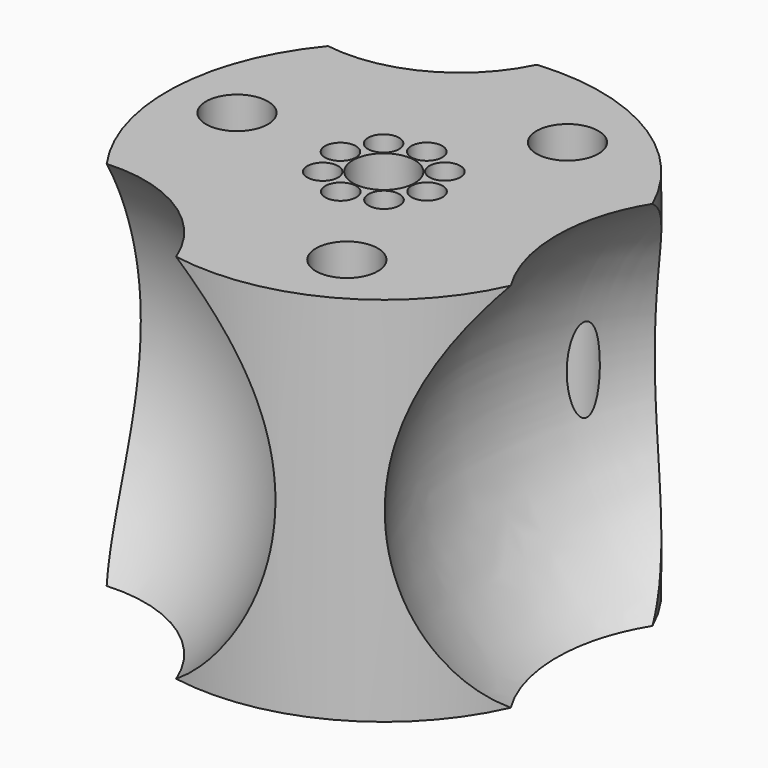
from build123d import *

# Parameters (mm, degrees)
F0_R          = 44.45
F0_R_2        = 16.51
F1_DEPTH      = 38.1
F1_DEPTH_BACK = 38.1
F8_R          = 3.175
F8_R_2        = 1.9685
F9_DEPTH      = 48.26
F10_R         = 6.35
F11_DEPTH     = 7.62
F12_R         = 3.429
F13_DEPTH     = 68.58
F14_R         = 6.35
F15_DEPTH     = 76.2


# Not quite as in the source:
# - a feature names something its author has since deleted; it is built from what else it names


with BuildPart() as f1:
    # F0 (on Top) → F1 (new body, two sides)
    with BuildSketch(Plane.XY) as f1_sk:
        with Locations((-96.7949852347, 47.625)):
            Circle(F0_R)
        with Locations((-96.7949852347, 47.625)):
            Circle(F0_R_2, mode=Mode.SUBTRACT)
        with Locations((-96.7949852347, 47.625)):
            Circle(F0_R_2)
        with BuildLine():
            ThreePointArc((-88.1051627648, 52.1100670498), (-87.4115771175, 50.37826953), (-87.0594782396, 48.5462733292))
            ThreePointArc((-87.0594782396, 48.5462733292), (-85.6757800173, 47.965243489), (-85.103715896, 46.5778145407))
            ThreePointArc((-85.103715896, 46.5778145407), (-85.8323827306, 45.0488259953), (-87.478931514, 44.6517889292))
            ThreePointArc((-87.478931514, 44.6517889292), (-88.2130581693, 42.9367840447), (-89.2595036018, 41.3923956038))
            ThreePointArc((-89.2595036018, 41.3923956038), (-88.839336444, 40.7569162622), (-88.6919210429, 40.0094919292))
            ThreePointArc((-88.6919210429, 40.0094919292), (-90.1000831422, 38.1224270954), (-92.309918185, 38.9351775301))
            ThreePointArc((-92.309918185, 38.9351775301), (-94.0417157047, 38.2415918827), (-95.8737119056, 37.8894930048))
            ThreePointArc((-95.8737119056, 37.8894930048), (-98.0529677671, 35.9450498204), (-99.7681963056, 38.3089462792))
            ThreePointArc((-99.7681963056, 38.3089462792), (-101.48320119, 39.0430729345), (-103.0275896309, 40.089518367))
            ThreePointArc((-103.0275896309, 40.089518367), (-105.9434851899, 40.2555560033), (-105.4848077047, 43.1399329502))
            ThreePointArc((-105.4848077047, 43.1399329502), (-106.178393352, 44.87173047), (-106.5304922299, 46.7037266708))
            ThreePointArc((-106.5304922299, 46.7037266708), (-108.4749354144, 48.8829825323), (-106.1110389555, 50.5982110708))
            ThreePointArc((-106.1110389555, 50.5982110708), (-105.3769123002, 52.3132159553), (-104.3304668677, 53.8576043962))
            ThreePointArc((-104.3304668677, 53.8576043962), (-104.1644292314, 56.7734999551), (-101.2800522845, 56.3148224699))
            ThreePointArc((-101.2800522845, 56.3148224699), (-99.5482547647, 57.0084081173), (-97.7162585639, 57.3605069952))
            ThreePointArc((-97.7162585639, 57.3605069952), (-95.7414309138, 59.3162590358), (-93.7792997754, 57.3477693387))
            ThreePointArc((-93.7792997754, 57.3477693387), (-93.7899471678, 57.1433056087), (-93.8217741639, 56.9410537208))
            ThreePointArc((-93.8217741639, 56.9410537208), (-92.1067692795, 56.2069270655), (-90.5623808386, 55.160481633))
            ThreePointArc((-90.5623808386, 55.160481633), (-88.4202847093, 55.5757742752), (-87.210977164, 53.7595641919))
            ThreePointArc((-87.210977164, 53.7595641919), (-87.4489020941, 52.8214265806), (-88.1051627648, 52.1100670498))
        make_face(mode=Mode.SUBTRACT)
        with BuildLine():
            ThreePointArc((-87.478931514, 44.6517889292), (-89.0293967369, 46.7886116136), (-87.0594782396, 48.5462733292))
            ThreePointArc((-87.0594782396, 48.5462733292), (-87.4115771175, 50.37826953), (-88.1051627648, 52.1100670498))
            ThreePointArc((-88.1051627648, 52.1100670498), (-90.7124690483, 52.524684387), (-90.5623808386, 55.160481633))
            ThreePointArc((-90.5623808386, 55.160481633), (-92.1067692795, 56.2069270655), (-93.8217741639, 56.9410537208))
            ThreePointArc((-93.8217741639, 56.9410537208), (-95.9585968484, 55.3905884978), (-97.7162585639, 57.3605069952))
            ThreePointArc((-97.7162585639, 57.3605069952), (-99.5482547647, 57.0084081173), (-101.2800522845, 56.3148224699))
            ThreePointArc((-101.2800522845, 56.3148224699), (-101.0424845928, 55.8008459714), (-100.9610494266, 55.2405080708))
            ThreePointArc((-100.9610494266, 55.2405080708), (-102.1821250936, 53.4194234719), (-104.3304668677, 53.8576043962))
            ThreePointArc((-104.3304668677, 53.8576043962), (-105.3769123002, 52.3132159553), (-106.1110389555, 50.5982110708))
            ThreePointArc((-106.1110389555, 50.5982110708), (-104.988766028, 49.9120186247), (-104.5492545734, 48.6721854593))
            ThreePointArc((-104.5492545734, 48.6721854593), (-105.1303256251, 47.2757495806), (-106.5304922299, 46.7037266708))
            ThreePointArc((-106.5304922299, 46.7037266708), (-106.178393352, 44.87173047), (-105.4848077047, 43.1399329502))
            ThreePointArc((-105.4848077047, 43.1399329502), (-103.4723556943, 43.221010878), (-102.4419933055, 41.4904358081))
            ThreePointArc((-102.4419933055, 41.4904358081), (-102.5942832222, 40.7312433534), (-103.0275896309, 40.089518367))
            ThreePointArc((-103.0275896309, 40.089518367), (-101.48320119, 39.0430729345), (-99.7681963056, 38.3089462792))
            ThreePointArc((-99.7681963056, 38.3089462792), (-97.6377069641, 39.8600832689), (-95.8736706941, 37.9022306613))
            ThreePointArc((-95.8736706941, 37.9022306613), (-95.873680997, 37.8958617997), (-95.8737119056, 37.8894930048))
            ThreePointArc((-95.8737119056, 37.8894930048), (-94.0417157047, 38.2415918827), (-92.309918185, 38.9351775301))
            ThreePointArc((-92.309918185, 38.9351775301), (-91.8953008477, 41.5424838136), (-89.2595036018, 41.3923956038))
            ThreePointArc((-89.2595036018, 41.3923956038), (-88.2130581693, 42.9367840447), (-87.478931514, 44.6517889292))
        make_face()
    extrude(amount=F1_DEPTH)
    extrude(f1_sk.sketch, amount=-F1_DEPTH_BACK)

    # F2 (on Top) → F3 (revolve, cut)
    with BuildSketch(Plane.XY):
        with BuildLine():
            Line((-32.5839432458, 95.377), (-32.5839432458, 47.625))
            Line((-32.5839432458, 47.625), (-32.5839432458, -0.127))
            Line((-32.5839432458, -0.127), (-32.5839432458, -9.525))
            ThreePointArc((-32.5839432458, -9.525), (15.1680567542, 47.625), (-32.5839432458, 104.775))
            Line((-32.5839432458, 104.775), (-32.5839432458, 95.377))
        make_face()
    revolve(axis=Axis((-32.5839432458, 19.05, 0), (0, -1, 0)), mode=Mode.SUBTRACT)

    # F4 (on Top) → F5 (revolve, cut)
    with BuildSketch(Plane.XY):
        with BuildLine():
            Line((-88.4089947582, -28.0660327723), (-131.1163690465, -6.7040645718))
            Line((-131.1163690465, -6.7040645718), (-173.8237433348, 14.6579036287))
            ThreePointArc((-173.8237433348, 14.6579036287), (-152.478337247, -49.4114388601), (-88.4089947582, -28.0660327723))
        make_face()
    revolve(axis=Axis((-152.4700561907, 3.9769195285, 0), (-0.894357813, 0.4473523245, 0)), mode=Mode.SUBTRACT)

    # F6 (on Top) → F7 (revolve, cut)
    with BuildSketch(Plane.XY):
        with BuildLine():
            ThreePointArc((-83.0436281881, 123.89609931), (-146.068020162, 148.1537377837), (-170.3256586357, 85.1293458098))
            Line((-170.3256586357, 85.1293458098), (-126.6846434119, 104.5127225599))
            Line((-126.6846434119, 104.5127225599), (-83.0436281881, 123.89609931))
        make_face()
    revolve(axis=Axis((-148.5051510238, 94.8210341849, 0), (0.9139096839, 0.4059175898, 0)), mode=Mode.SUBTRACT)

    # F8 (on face) → F9 (cut)
    with BuildSketch(Plane.XY.offset(38.1)):
        with Locations((-102.9295494266, 55.2405080708)):
            Circle(F8_R)
        with Locations((-102.9295494266, 55.2405080708)):
            Circle(F8_R_2, mode=Mode.SUBTRACT)
        with Locations((-95.7477997754, 57.3477693387)):
            Circle(F8_R)
        with Locations((-95.7477997754, 57.3477693387)):
            Circle(F8_R_2, mode=Mode.SUBTRACT)
        with Locations((-89.179477164, 53.7595641919)):
            Circle(F8_R)
        with Locations((-89.179477164, 53.7595641919)):
            Circle(F8_R_2, mode=Mode.SUBTRACT)
        with Locations((-87.072215896, 46.5778145407)):
            Circle(F8_R)
        with Locations((-87.072215896, 46.5778145407)):
            Circle(F8_R_2, mode=Mode.SUBTRACT)
        with Locations((-90.6604210429, 40.0094919292)):
            Circle(F8_R)
        with Locations((-90.6604210429, 40.0094919292)):
            Circle(F8_R_2, mode=Mode.SUBTRACT)
        with Locations((-97.8421706941, 37.9022306613)):
            Circle(F8_R)
        with BuildLine():
            ThreePointArc((-95.8736706941, 37.9022306613), (-95.873680997, 37.8958617997), (-95.8737119056, 37.8894930048))
            ThreePointArc((-95.8737119056, 37.8894930048), (-99.8106603912, 37.9085995228), (-95.8736706941, 37.9022306613))
        make_face(mode=Mode.SUBTRACT)
        with Locations((-104.4104933055, 41.4904358081)):
            Circle(F8_R)
        with Locations((-104.4104933055, 41.4904358081)):
            Circle(F8_R_2, mode=Mode.SUBTRACT)
        with Locations((-106.5177545734, 48.6721854593)):
            Circle(F8_R)
        with Locations((-106.5177545734, 48.6721854593)):
            Circle(F8_R_2, mode=Mode.SUBTRACT)
    extrude(amount=-F9_DEPTH, mode=Mode.SUBTRACT)

    # F10 (on face) → F11 (cut)
    with BuildSketch(Plane.XY.offset(38.1)):
        with Locations((-96.7949852347, 47.625)):
            Circle(F10_R)
    extrude(amount=-F11_DEPTH, mode=Mode.SUBTRACT)

    # F12 (on face) → F13 (cut, through all)
    with BuildSketch(Plane.XY.offset(30.48)):
        with Locations((-96.7949852347, 47.625)):
            Circle(F12_R)
    extrude(amount=-F13_DEPTH, mode=Mode.SUBTRACT)

    # F14 (on face) → F15 (cut, through all)
    with BuildSketch(Plane.XY.offset(38.1)):
        with Locations((-127.8890646346, 48.8640254414)):
            Circle(F14_R)
        with BuildLine():
            ThreePointArc((-76.7834769385, 79.3022345884), (-85.5434026681, 77.325191035), (-83.5663591148, 68.5652653054))
            Line((-83.5663591148, 68.5652653054), (-76.7834769385, 79.3022345884))
        make_face()
        with BuildLine():
            Line((-76.7834769385, 79.3022345884), (-83.5663591148, 68.5652653054))
            ThreePointArc((-83.5663591148, 68.5652653054), (-77.1100486093, 68.3723584434), (-73.8249180267, 73.9337499469))
            ThreePointArc((-73.8249180267, 73.9337499469), (-74.6135265232, 76.9986193642), (-76.7834769385, 79.3022345884))
        make_face()
        with Locations((-82.3209730429, 20.0772246117)):
            Circle(F14_R)
    extrude(amount=-F15_DEPTH, mode=Mode.SUBTRACT)


solid = f1.part
